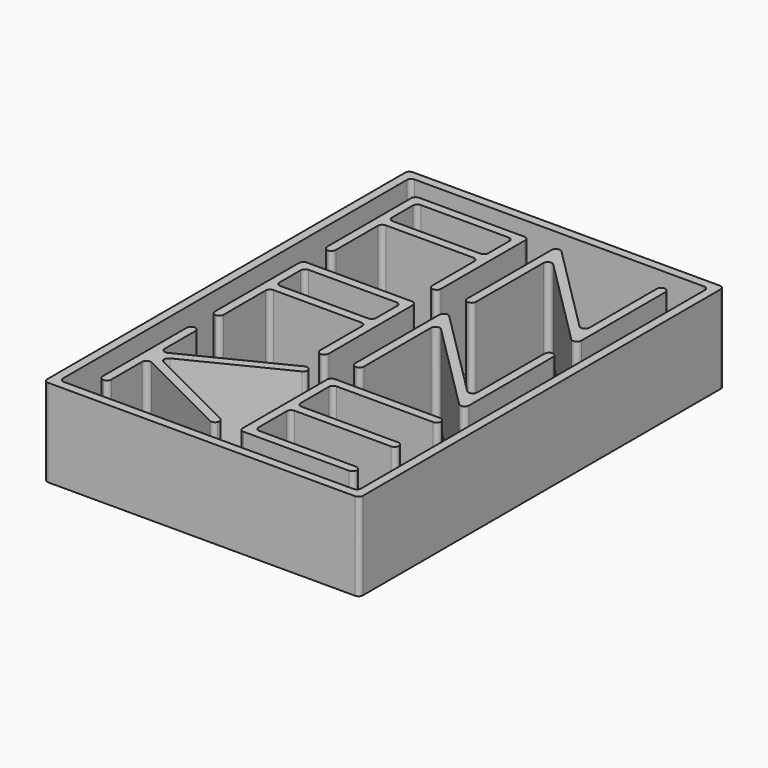
from build123d import *

# Parameters (mm, degrees)
F1_W     = 18
F1_H     = 26
F1_W_2   = 17
F1_H_2   = 25
F2_DEPTH = 5
F1_W_3   = 6
F1_H_3   = 2.5
F1_W_4   = 5.5
F1_H_4   = 2
F3_R     = 0.25
F4_R     = 0.24999
F5_R     = 0.24999
F6_R     = 0.24999
F7_R     = 0.24999
F8_R     = 0.24999
F9_R     = 0.24999


# Not quite as in the source:
# - a fillet or chamfer is up to 0.001 mm smaller than in the source, because OpenCascade refuses the exact size


with BuildPart() as f2:
    # F1 (on face) → F2 (new body)
    with BuildSketch(Plane.XY):
        Rectangle(F1_W, F1_H)
        Rectangle(F1_W_2, F1_H_2, mode=Mode.SUBTRACT)
    extrude(amount=F2_DEPTH)

    # F3
    f3_edges = [f2.edges().sort_by_distance(p)[0] for p in [
        (9, 13, 2.5),
        (-9, 13, 2.5),
        (8.5, 12.5, 2.5),
        (-8.5, 12.5, 2.5),
        (9, -13, 2.5),
        (-9, -13, 2.5),
        (8.5, -12.5, 2.5),
        (-8.5, -12.5, 2.5),
    ]]
    fillet(f3_edges, radius=F3_R)


with BuildPart() as f2b:
    # F1 (on face) → F2, piece 2 (new body)
    with BuildSketch(Plane.XY):
        Polygon((-0.75, 5), (-0.75, 11.25), (-7.25, 11.25), (-7.25, 5), (-7.25, 4.75), (-6.75, 4.75), (-6.75, 5), (-6.75, 8.25), (-1.25, 8.25), (-1.25, 5), (-1, 5), align=None)
        with Locations((-4, 9.75)):
            Rectangle(F1_W_3, F1_H_3, mode=Mode.SUBTRACT)
        Polygon((-0.75, 4.75), (-0.75, 5), (-1, 5), (-1.25, 5), (-1.25, 4.75), align=None)
        with Locations((-4, 9.75)):
            Rectangle(F1_W_3, F1_H_3)
        with Locations((-4, 9.75)):
            Rectangle(F1_W_4, F1_H_4, mode=Mode.SUBTRACT)
    extrude(amount=F2_DEPTH)

    # F4 (radius 0.25 in the source; OpenCascade refuses exactly that, so slightly less here)
    f4_edges = [f2b.edges().sort_by_distance(p)[0] for p in [
        (-6.75, 10.75, 2.5),
        (-6.75, 8.25, 2.5),
        (-6.75, 4.75, 2.5),
        (-0.75, 4.75, 2.5),
        (-7.25, 4.75, 2.5),
        (-1.25, 4.75, 2.5),
        (-0.75, 11.25, 2.5),
        (-1.25, 10.75, 2.5),
        (-1.25, 8.25, 2.5),
        (-7.25, 11.25, 2.5),
        (-1.25, 8.75, 2.5),
        (-6.75, 8.75, 2.5),
    ]]
    fillet(f4_edges, radius=F4_R)


with BuildPart() as f2c:
    # F1 (on face) → F2, piece 3 (new body)
    with BuildSketch(Plane.XY):
        Polygon((6.75, 11), (6.75, 5.6035533906), (0.75, 11.6035533906), (0.75, 5), (0.75, 4.75), (1.25, 4.75), (1.25, 5), (1.25, 10.3964466094), (7.25, 4.3964466094), (7.25, 11), (7.25, 11.25), (6.75, 11.25), align=None)
    extrude(amount=F2_DEPTH)

    # F5 (radius 0.25 in the source; OpenCascade refuses exactly that, so slightly less here)
    f5_edges = [f2c.edges().sort_by_distance(p)[0] for p in [
        (7.25, 11.25, 2.5),
        (6.75, 11.25, 2.5),
        (0.75, 11.603553, 2.5),
        (7.25, 4.396447, 2.5),
        (1.25, 4.75, 2.5),
        (0.75, 4.75, 2.5),
        (6.75, 5.603553, 2.5),
        (1.25, 10.396447, 2.5),
    ]]
    fillet(f5_edges, radius=F5_R)


with BuildPart() as f2d:
    # F1 (on face) → F2, piece 4 (new body)
    with BuildSketch(Plane.XY):
        Polygon((1.25, 2.3964466094), (7.25, -3.6035533906), (7.25, 3), (7.25, 3.25), (6.75, 3.25), (6.75, 3), (6.75, -2.3964466094), (0.75, 3.6035533906), (0.75, -3), (0.75, -3.25), (1.25, -3.25), (1.25, -3), align=None)
    extrude(amount=F2_DEPTH)

    # F6 (radius 0.25 in the source; OpenCascade refuses exactly that, so slightly less here)
    f6_edges = [f2d.edges().sort_by_distance(p)[0] for p in [
        (7.25, -3.603553, 2.5),
        (1.25, -3.25, 2.5),
        (0.75, -3.25, 2.5),
        (7.25, 3.25, 2.5),
        (1.25, 2.396447, 2.5),
        (0.75, 3.603553, 2.5),
        (6.75, 3.25, 2.5),
        (6.75, -2.396447, 2.5),
    ]]
    fillet(f6_edges, radius=F6_R)


with BuildPart() as f2e:
    # F1 (on face) → F2, piece 5 (new body)
    with BuildSketch(Plane.XY):
        Polygon((-0.75, 3.25), (-7.25, 3.25), (-7.25, -3), (-7.25, -3.25), (-6.75, -3.25), (-6.75, -3), (-6.75, 0.25), (-1.25, 0.25), (-1.25, -3), (-1.25, -3.25), (-0.75, -3.25), (-0.75, -3), align=None)
        with Locations((-4, 1.75)):
            Rectangle(F1_W_3, F1_H_3, mode=Mode.SUBTRACT)
        with Locations((-4, 1.75)):
            Rectangle(F1_W_3, F1_H_3)
        with Locations((-4, 1.75)):
            Rectangle(F1_W_4, F1_H_4, mode=Mode.SUBTRACT)
    extrude(amount=F2_DEPTH)

    # F7 (radius 0.25 in the source; OpenCascade refuses exactly that, so slightly less here)
    f7_edges = [f2e.edges().sort_by_distance(p)[0] for p in [
        (-0.75, 3.25, 2.5),
        (-7.25, 3.25, 2.5),
        (-7.25, -3.25, 2.5),
        (-1.25, -3.25, 2.5),
        (-1.25, 0.75, 2.5),
        (-6.75, 0.75, 2.5),
        (-1.25, 0.25, 2.5),
        (-6.75, 0.25, 2.5),
        (-6.75, -3.25, 2.5),
        (-6.75, 2.75, 2.5),
        (-1.25, 2.75, 2.5),
        (-0.75, -3.25, 2.5),
    ]]
    fillet(f7_edges, radius=F7_R)


with BuildPart() as f2f:
    # F1 (on face) → F2, piece 6 (new body)
    with BuildSketch(Plane.XY):
        Polygon((0.75, -4.75), (0.75, -11.25), (7, -11.25), (7.25, -11.25), (7.25, -10.75), (7, -10.75), (1.25, -10.75), (1.25, -8.25), (7.25, -8.25), (7.25, -7.75), (1.25, -7.75), (1.25, -5.25), (7, -5.25), (7.25, -5.25), (7.25, -4.75), (7, -4.75), align=None)
    extrude(amount=F2_DEPTH)

    # F8 (radius 0.25 in the source; OpenCascade refuses exactly that, so slightly less here)
    f8_edges = [f2f.edges().sort_by_distance(p)[0] for p in [
        (1.25, -5.25, 2.5),
        (7.25, -5.25, 2.5),
        (7.25, -4.75, 2.5),
        (7.25, -8.25, 2.5),
        (7.25, -7.75, 2.5),
        (1.25, -8.25, 2.5),
        (7.25, -11.25, 2.5),
        (7.25, -10.75, 2.5),
        (0.75, -11.25, 2.5),
        (1.25, -10.75, 2.5),
        (1.25, -7.75, 2.5),
        (0.75, -4.75, 2.5),
    ]]
    fillet(f8_edges, radius=F8_R)


with BuildPart() as f2g:
    # F1 (on face) → F2, piece 7 (new body)
    with BuildSketch(Plane.XY):
        Polygon((-6.75, -4.75), (-7.25, -4.75), (-7.25, -11.25), (-6.75, -11.25), (-6.75, -8.4045084972), (-0.6118033989, -11.4736067977), (-0.3881966011, -11.0263932023), (-6.4409830056, -8), (-0.3881966011, -4.9736067977), (-0.6118033989, -4.5263932023), (-6.75, -7.5954915028), align=None)
    extrude(amount=F2_DEPTH)

    # F9 (radius 0.25 in the source; OpenCascade refuses exactly that, so slightly less here)
    f9_edges = [f2g.edges().sort_by_distance(p)[0] for p in [
        (-6.440983, -8, 2.5),
        (-0.388197, -4.973607, 2.5),
        (-0.611803, -4.526393, 2.5),
        (-0.388197, -11.026393, 2.5),
        (-6.75, -11.25, 2.5),
        (-7.25, -11.25, 2.5),
        (-6.75, -4.75, 2.5),
        (-0.611803, -11.473607, 2.5),
        (-6.75, -8.404508, 2.5),
        (-6.75, -7.595492, 2.5),
        (-7.25, -4.75, 2.5),
    ]]
    fillet(f9_edges, radius=F9_R)


solid = Compound([f2.part, f2b.part, f2c.part, f2d.part, f2e.part, f2f.part, f2g.part])
